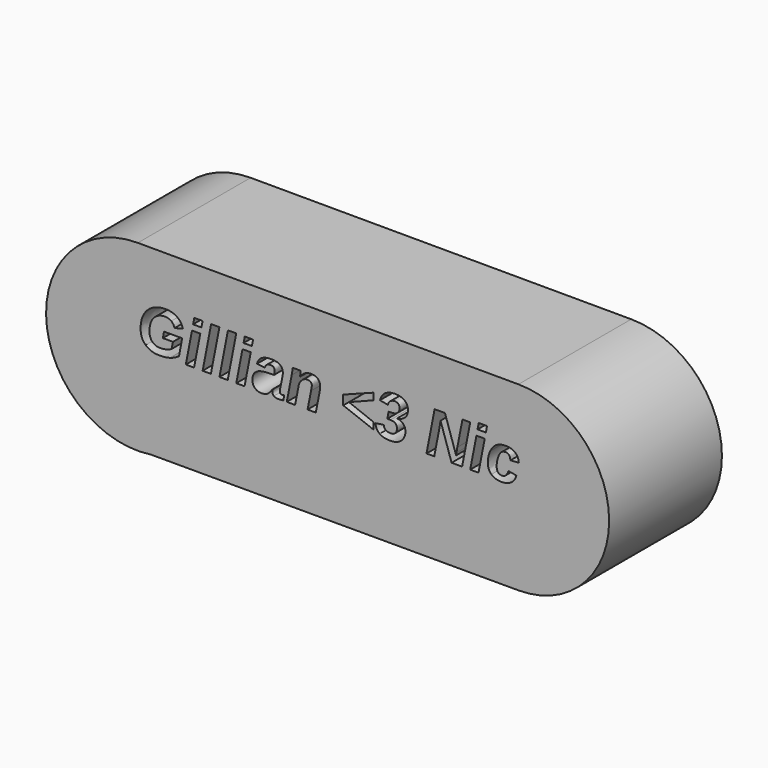
from build123d import *

# Parameters (mm, degrees)
F1_DEPTH = 25.4


with BuildPart() as f1:
    # F0 (on Front) → F1 (new body)
    with BuildSketch(Plane.XZ):
        with BuildLine():
            Line((28.869589976, 36.934029669), (-39.7119261324, 37.0742306113))
            ThreePointArc((-39.7119261324, 37.0742306113), (-56.2022137715, 19.4003067851), (-37.3673066497, 4.2496155947))
            Line((-37.3673066497, 4.2496155947), (28.869589976, 4.2496155947))
            ThreePointArc((28.869589976, 4.2496155947), (45.2117970132, 20.5918226319), (28.869589976, 36.934029669))
        make_face()
        with BuildLine():
            add(Edge.make_bspline(
                [(-33.9471180294, 20.7070778912), (-34.7784034926, 20.475170562), (-35.8015240626, 20.475170562)],
                knots=[0, 0, 0, 1, 1, 1], degree=2))
            add(Edge.make_bspline(
                [(-35.8015240626, 20.475170562), (-37.4010025537, 20.475170562), (-38.3064642581, 21.3192450322)],
                knots=[0, 0, 0, 1, 1, 1], degree=2))
            add(Edge.make_bspline(
                [(-38.3064642581, 21.3192450322), (-39.2119259626, 22.1633195025), (-39.2119259626, 23.6826535489)],
                knots=[0, 0, 0, 1, 1, 1], degree=2))
            add(Edge.make_bspline(
                [(-39.2119259626, 23.6826535489), (-39.2119259626, 25.0144154908), (-38.6551778524, 26.048619867)],
                knots=[0, 0, 0, 1, 1, 1], degree=2))
            add(Edge.make_bspline(
                [(-38.6551778524, 26.048619867), (-38.0984297422, 27.0828242432), (-37.0778669736, 27.6395723534)],
                knots=[0, 0, 0, 1, 1, 1], degree=2))
            add(Edge.make_bspline(
                [(-37.0778669736, 27.6395723534), (-36.0573042051, 28.1963204635), (-34.7255422631, 28.1963204635)],
                knots=[0, 0, 0, 1, 1, 1], degree=2))
            add(Edge.make_bspline(
                [(-34.7255422631, 28.1963204635), (-33.5114391867, 28.1963204635), (-32.6929427307, 27.6472457576)],
                knots=[0, 0, 0, 1, 1, 1], degree=2))
            add(Edge.make_bspline(
                [(-32.6929427307, 27.6472457576), (-31.8744462747, 27.0981710517), (-31.593088118, 26.1125649026)],
                knots=[0, 0, 0, 1, 1, 1], degree=2))
            Line((-31.593088118, 26.1125649026), (-33.0953701549, 25.6964958708))
            add(Edge.make_bspline(
                [(-33.0953701549, 25.6964958708), (-33.2505434414, 26.2984318062), (-33.6921904874, 26.6292407905)],
                knots=[0, 0, 0, 1, 1, 1], degree=2))
            add(Edge.make_bspline(
                [(-33.6921904874, 26.6292407905), (-34.1338375335, 26.9600497748), (-34.8108023106, 26.9600497748)],
                knots=[0, 0, 0, 1, 1, 1], degree=2))
            add(Edge.make_bspline(
                [(-34.8108023106, 26.9600497748), (-35.6582871828, 26.9600497748), (-36.297737539, 26.560180152)],
                knots=[0, 0, 0, 1, 1, 1], degree=2))
            add(Edge.make_bspline(
                [(-36.297737539, 26.560180152), (-36.9371878953, 26.1603105292), (-37.2782280853, 25.4253689198)],
                knots=[0, 0, 0, 1, 1, 1], degree=2))
            add(Edge.make_bspline(
                [(-37.2782280853, 25.4253689198), (-37.6192682753, 24.6904273103), (-37.6192682753, 23.7303991755)],
                knots=[0, 0, 0, 1, 1, 1], degree=2))
            add(Edge.make_bspline(
                [(-37.6192682753, 23.7303991755), (-37.6192682753, 22.7823074473), (-37.1102657917, 22.2409061457)],
                knots=[0, 0, 0, 1, 1, 1], degree=2))
            add(Edge.make_bspline(
                [(-37.1102657917, 22.2409061457), (-36.6012633081, 21.6995048441), (-35.6736339913, 21.6995048441)],
                knots=[0, 0, 0, 1, 1, 1], degree=2))
            add(Edge.make_bspline(
                [(-35.6736339913, 21.6995048441), (-35.0989812712, 21.6995048441), (-34.5550221681, 21.8384787215)],
                knots=[0, 0, 0, 1, 1, 1], degree=2))
            add(Edge.make_bspline(
                [(-34.5550221681, 21.8384787215), (-34.0110630651, 21.9774525989), (-33.6273928513, 22.2110651291)],
                knots=[0, 0, 0, 1, 1, 1], degree=2))
            Line((-33.6273928513, 22.2110651291), (-33.3835491155, 23.4268734064))
            Line((-33.3835491155, 23.4268734064), (-35.2047037301, 23.4268734064))
            Line((-35.2047037301, 23.4268734064), (-34.9983744151, 24.5352540239))
            Line((-34.9983744151, 24.5352540239), (-31.7260937921, 24.5352540239))
            Line((-31.7260937921, 24.5352540239), (-32.2853997037, 21.5085223377))
            add(Edge.make_bspline(
                [(-32.2853997037, 21.5085223377), (-33.1158325663, 20.9389852204), (-33.9471180294, 20.7070778912)],
                knots=[0, 0, 0, 1, 1, 1], degree=2))
        make_face(mode=Mode.SUBTRACT)
        Polygon((-29.579245796, 20.575777418), (-31.0712966273, 20.575777418), (-29.9509796031, 26.3410618299), (-28.453813169, 26.3410618299), align=None, mode=Mode.SUBTRACT)
        Polygon((-26.5473985069, 20.575777418), (-28.0394493382, 20.575777418), (-26.5047684832, 28.4844994241), (-25.0058968481, 28.4844994241), align=None, mode=Mode.SUBTRACT)
        Polygon((-20.4837039287, 20.575777418), (-21.97575476, 20.575777418), (-20.8554377358, 26.3410618299), (-19.3582713017, 26.3410618299), align=None, mode=Mode.SUBTRACT)
        Polygon((-23.5155512178, 20.575777418), (-25.0076020491, 20.575777418), (-23.4729211941, 28.4844994241), (-21.974049559, 28.4844994241), align=None, mode=Mode.SUBTRACT)
        with BuildLine():
            add(Edge.make_bspline(
                [(-13.9075964651, 20.5382629971), (-14.1369459929, 20.5229161886), (-14.3756741259, 20.5229161886)],
                knots=[0, 0, 0, 1, 1, 1], degree=2))
            add(Edge.make_bspline(
                [(-14.3756741259, 20.5229161886), (-14.9094020232, 20.5229161886), (-15.1967283833, 20.746297513)],
                knots=[0, 0, 0, 1, 1, 1], degree=2))
            add(Edge.make_bspline(
                [(-15.1967283833, 20.746297513), (-15.4840547434, 20.9696788375), (-15.4840547434, 21.3380022427)],
                knots=[0, 0, 0, 1, 1, 1], degree=2))
            add(Edge.make_bspline(
                [(-15.4840547434, 21.3380022427), (-15.4840547434, 21.5358055529), (-15.4584767291, 21.6790424327)],
                knots=[0, 0, 0, 1, 1, 1], degree=2))
            Line((-15.4584767291, 21.6790424327), (-15.4908755472, 21.6790424327))
            add(Edge.make_bspline(
                [(-15.4908755472, 21.6790424327), (-15.9376381961, 20.986730847), (-16.3750222397, 20.7275403026)],
                knots=[0, 0, 0, 1, 1, 1], degree=2))
            add(Edge.make_bspline(
                [(-16.3750222397, 20.7275403026), (-16.8124062834, 20.4683497582), (-17.439920233, 20.4683497582)],
                knots=[0, 0, 0, 1, 1, 1], degree=2))
            add(Edge.make_bspline(
                [(-17.439920233, 20.4683497582), (-18.1867982491, 20.4683497582), (-18.631855697, 20.9134072061)],
                knots=[0, 0, 0, 1, 1, 1], degree=2))
            add(Edge.make_bspline(
                [(-18.631855697, 20.9134072061), (-19.076913145, 21.3584646541), (-19.076913145, 22.0575970436)],
                knots=[0, 0, 0, 1, 1, 1], degree=2))
            add(Edge.make_bspline(
                [(-19.076913145, 22.0575970436), (-19.076913145, 23.0432031927), (-18.3973905664, 23.5470900734)],
                knots=[0, 0, 0, 1, 1, 1], degree=2))
            add(Edge.make_bspline(
                [(-18.3973905664, 23.5470900734), (-17.7178679878, 24.0509769541), (-16.1934183386, 24.0765549683)],
                knots=[0, 0, 0, 1, 1, 1], degree=2))
            Line((-16.1934183386, 24.0765549683), (-15.1754133714, 24.0936069778))
            add(Edge.make_bspline(
                [(-15.1754133714, 24.0936069778), (-15.0645753097, 24.598346459), (-15.0645753097, 24.7910341664)],
                knots=[0, 0, 0, 1, 1, 1], degree=2))
            add(Edge.make_bspline(
                [(-15.0645753097, 24.7910341664), (-15.0645753097, 25.4731145464), (-15.7398348859, 25.4731145464)],
                knots=[0, 0, 0, 1, 1, 1], degree=2))
            add(Edge.make_bspline(
                [(-15.7398348859, 25.4731145464), (-16.2411639652, 25.4731145464), (-16.486712902, 25.2787216381)],
                knots=[0, 0, 0, 1, 1, 1], degree=2))
            add(Edge.make_bspline(
                [(-16.486712902, 25.2787216381), (-16.7322618388, 25.0843287298), (-16.8226374891, 24.7160053246)],
                knots=[0, 0, 0, 1, 1, 1], degree=2))
            Line((-16.8226374891, 24.7160053246), (-18.22431267, 24.8814098167))
            add(Edge.make_bspline(
                [(-18.22431267, 24.8814098167), (-18.0418561683, 25.6487502442), (-17.405816214, 26.048619867)],
                knots=[0, 0, 0, 1, 1, 1], degree=2))
            add(Edge.make_bspline(
                [(-17.405816214, 26.048619867), (-16.7697762597, 26.4484894898), (-15.7142568716, 26.4484894898)],
                knots=[0, 0, 0, 1, 1, 1], degree=2))
            add(Edge.make_bspline(
                [(-15.7142568716, 26.4484894898), (-14.610991857, 26.4484894898), (-14.0968737705, 26.0597036732)],
                knots=[0, 0, 0, 1, 1, 1], degree=2))
            add(Edge.make_bspline(
                [(-14.0968737705, 26.0597036732), (-13.5827556841, 25.6709178566), (-13.5827556841, 24.8762942139)],
                knots=[0, 0, 0, 1, 1, 1], degree=2))
            add(Edge.make_bspline(
                [(-13.5827556841, 24.8762942139), (-13.5827556841, 24.6784909037), (-13.7106457554, 24.0390405474)],
                knots=[0, 0, 0, 1, 1, 1], degree=2))
            Line((-13.7106457554, 24.0390405474), (-14.0892003663, 22.1582038996))
            add(Edge.make_bspline(
                [(-14.0892003663, 22.1582038996), (-14.13183039, 21.9194757666), (-14.13183039, 21.7745336859)],
                knots=[0, 0, 0, 1, 1, 1], degree=2))
            add(Edge.make_bspline(
                [(-14.13183039, 21.7745336859), (-14.13183039, 21.6466436146), (-14.0781165601, 21.5775829761)],
                knots=[0, 0, 0, 1, 1, 1], degree=2))
            add(Edge.make_bspline(
                [(-14.0781165601, 21.5775829761), (-14.0244027302, 21.5085223377), (-13.9553420917, 21.4761235196)],
                knots=[0, 0, 0, 1, 1, 1], degree=2))
            add(Edge.make_bspline(
                [(-13.9553420917, 21.4761235196), (-13.8862814532, 21.4437247016), (-13.8172208147, 21.4360512973)],
                knots=[0, 0, 0, 1, 1, 1], degree=2))
            add(Edge.make_bspline(
                [(-13.8172208147, 21.4360512973), (-13.7481601763, 21.428377893), (-13.7106457554, 21.428377893)],
                knots=[0, 0, 0, 1, 1, 1], degree=2))
            add(Edge.make_bspline(
                [(-13.7106457554, 21.428377893), (-13.5503568661, 21.428377893), (-13.3798367711, 21.4658923139)],
                knots=[0, 0, 0, 1, 1, 1], degree=2))
            Line((-13.3798367711, 21.4658923139), (-13.4548656129, 20.6405750541))
            add(Edge.make_bspline(
                [(-13.4548656129, 20.6405750541), (-13.6782469373, 20.5536098057), (-13.9075964651, 20.5382629971)],
                knots=[0, 0, 0, 1, 1, 1], degree=2))
        make_face(mode=Mode.SUBTRACT)
        with BuildLine():
            Line((-7.6418355743, 20.575777418), (-9.1287708027, 20.575777418))
            Line((-9.1287708027, 20.575777418), (-8.4995516522, 23.7457459841))
            add(Edge.make_bspline(
                [(-8.4995516522, 23.7457459841), (-8.3614303752, 24.4073639526), (-8.3614303752, 24.6256296742)],
                knots=[0, 0, 0, 1, 1, 1], degree=2))
            add(Edge.make_bspline(
                [(-8.3614303752, 24.6256296742), (-8.3614303752, 25.3128256571), (-9.1714008265, 25.3128256571)],
                knots=[0, 0, 0, 1, 1, 1], degree=2))
            add(Edge.make_bspline(
                [(-9.1714008265, 25.3128256571), (-9.7085391257, 25.3128256571), (-10.1672381813, 24.8762942139)],
                knots=[0, 0, 0, 1, 1, 1], degree=2))
            add(Edge.make_bspline(
                [(-10.1672381813, 24.8762942139), (-10.6259372368, 24.4397627707), (-10.7435961024, 23.8054280173)],
                knots=[0, 0, 0, 1, 1, 1], degree=2))
            Line((-10.7435961024, 23.8054280173), (-11.371110052, 20.575777418))
            Line((-11.371110052, 20.575777418), (-12.8750972899, 20.575777418))
            Line((-12.8750972899, 20.575777418), (-11.9900979968, 25.109906744))
            add(Edge.make_bspline(
                [(-11.9900979968, 25.109906744), (-11.9048379493, 25.5310913787), (-11.7871790838, 26.3410618299)],
                knots=[0, 0, 0, 1, 1, 1], degree=2))
            Line((-11.7871790838, 26.3410618299), (-10.3599258886, 26.3410618299))
            add(Edge.make_bspline(
                [(-10.3599258886, 26.3410618299), (-10.3599258886, 26.2933162033), (-10.4102293166, 25.8934465806)],
                knots=[0, 0, 0, 1, 1, 1], degree=2))
            add(Edge.make_bspline(
                [(-10.4102293166, 25.8934465806), (-10.4605327447, 25.4935769578), (-10.4878159599, 25.3554556808)],
                knots=[0, 0, 0, 1, 1, 1], degree=2))
            Line((-10.4878159599, 25.3554556808), (-10.4707639504, 25.3554556808))
            add(Edge.make_bspline(
                [(-10.4707639504, 25.3554556808), (-10.0717469281, 25.9096459896), (-9.5891750592, 26.1765099383)],
                knots=[0, 0, 0, 1, 1, 1], degree=2))
            add(Edge.make_bspline(
                [(-9.5891750592, 26.1765099383), (-9.1066031904, 26.4433738869), (-8.4842048436, 26.4433738869)],
                knots=[0, 0, 0, 1, 1, 1], degree=2))
            add(Edge.make_bspline(
                [(-8.4842048436, 26.4433738869), (-7.6742343924, 26.4433738869), (-7.2632809634, 26.0537354699)],
                knots=[0, 0, 0, 1, 1, 1], degree=2))
            add(Edge.make_bspline(
                [(-7.2632809634, 26.0537354699), (-6.8523275345, 25.6640970528), (-6.8523275345, 24.9291554433)],
                knots=[0, 0, 0, 1, 1, 1], degree=2))
            add(Edge.make_bspline(
                [(-6.8523275345, 24.9291554433), (-6.8523275345, 24.7961497692), (-6.8898419554, 24.5054130073)],
                knots=[0, 0, 0, 1, 1, 1], degree=2))
            add(Edge.make_bspline(
                [(-6.8898419554, 24.5054130073), (-6.9273563763, 24.2146762453), (-6.9648707972, 24.0560925569)],
                knots=[0, 0, 0, 1, 1, 1], degree=2))
            Line((-6.9648707972, 24.0560925569), (-7.6418355743, 20.575777418))
        make_face(mode=Mode.SUBTRACT)
        Polygon((-28.2577150598, 27.3812344094), (-29.7548814939, 27.3812344094), (-29.5366157723, 28.4844994241), (-28.0377441372, 28.4844994241), align=None, mode=Mode.SUBTRACT)
        Polygon((-19.1621731925, 27.3812344094), (-20.6593396266, 27.3812344094), (-20.441073905, 28.4844994241), (-18.9422022699, 28.4844994241), align=None, mode=Mode.SUBTRACT)
        Polygon((2.7701214264, 21.2425109895), (-2.7018684222, 23.3262665504), (-2.7018684222, 25.041698706), (2.7701214264, 27.1254542669), (2.7701214264, 25.9096459896), (-1.6685166465, 24.1788670253), (2.7701214264, 22.451498463), align=None, mode=Mode.SUBTRACT)
        with BuildLine():
            Line((5.4728649321, 24.9939530794), (5.8616507487, 24.9939530794))
            add(Edge.make_bspline(
                [(5.8616507487, 24.9939530794), (6.6562743914, 24.9939530794), (7.0476180094, 25.3025944514)],
                knots=[0, 0, 0, 1, 1, 1], degree=2))
            add(Edge.make_bspline(
                [(7.0476180094, 25.3025944514), (7.4389616275, 25.6112358233), (7.4389616275, 26.1756573378)],
                knots=[0, 0, 0, 1, 1, 1], degree=2))
            add(Edge.make_bspline(
                [(7.4389616275, 26.1756573378), (7.4389616275, 26.5593275515), (7.233484913, 26.781003675)],
                knots=[0, 0, 0, 1, 1, 1], degree=2))
            add(Edge.make_bspline(
                [(7.233484913, 26.781003675), (7.0280081985, 27.0026797985), (6.601707961, 27.0026797985)],
                knots=[0, 0, 0, 1, 1, 1], degree=2))
            add(Edge.make_bspline(
                [(6.601707961, 27.0026797985), (5.6109862091, 27.0026797985), (5.339859258, 26.0221892523)],
                knots=[0, 0, 0, 1, 1, 1], degree=2))
            Line((5.339859258, 26.0221892523), (3.9160164648, 26.2984318062))
            add(Edge.make_bspline(
                [(3.9160164648, 26.2984318062), (4.4599755678, 28.1963204635), (6.6613899943, 28.1963204635)],
                knots=[0, 0, 0, 1, 1, 1], degree=2))
            add(Edge.make_bspline(
                [(6.6613899943, 28.1963204635), (7.7424873965, 28.1963204635), (8.3503915352, 27.7111907933)],
                knots=[0, 0, 0, 1, 1, 1], degree=2))
            add(Edge.make_bspline(
                [(8.3503915352, 27.7111907933), (8.9582956739, 27.226061123), (8.9582956739, 26.3632294423)],
                knots=[0, 0, 0, 1, 1, 1], degree=2))
            add(Edge.make_bspline(
                [(8.9582956739, 26.3632294423), (8.9582956739, 25.5310913787), (8.4407671856, 25.025499297)],
                knots=[0, 0, 0, 1, 1, 1], degree=2))
            add(Edge.make_bspline(
                [(8.4407671856, 25.025499297), (7.9232386972, 24.5199072153), (7.0331238014, 24.4397627707)],
                knots=[0, 0, 0, 1, 1, 1], degree=2))
            Line((7.0331238014, 24.4397627707), (7.0280081985, 24.4175951583))
            add(Edge.make_bspline(
                [(7.0280081985, 24.4175951583), (7.7476029994, 24.3067570966), (8.1235998089, 23.8881302634)],
                knots=[0, 0, 0, 1, 1, 1], degree=2))
            add(Edge.make_bspline(
                [(8.1235998089, 23.8881302634), (8.4995966183, 23.4695034302), (8.4995966183, 22.8027698587)],
                knots=[0, 0, 0, 1, 1, 1], degree=2))
            add(Edge.make_bspline(
                [(8.4995966183, 22.8027698587), (8.4995966183, 22.1428570911), (8.1534408255, 21.6014557894)],
                knots=[0, 0, 0, 1, 1, 1], degree=2))
            add(Edge.make_bspline(
                [(8.1534408255, 21.6014557894), (7.8072850326, 21.0600544878), (7.1780658821, 20.764202123)],
                knots=[0, 0, 0, 1, 1, 1], degree=2))
            add(Edge.make_bspline(
                [(7.1780658821, 20.764202123), (6.5488467316, 20.4683497582), (5.7337606775, 20.4683497582)],
                knots=[0, 0, 0, 1, 1, 1], degree=2))
            add(Edge.make_bspline(
                [(5.7337606775, 20.4683497582), (4.5298888068, 20.4683497582), (3.855481831, 20.9645632346)],
                knots=[0, 0, 0, 1, 1, 1], degree=2))
            add(Edge.make_bspline(
                [(3.855481831, 20.9645632346), (3.1810748553, 21.4607767111), (3.0958148078, 22.4037528364)],
                knots=[0, 0, 0, 1, 1, 1], degree=2))
            Line((3.0958148078, 22.4037528364), (4.5980968448, 22.6066717495))
            add(Edge.make_bspline(
                [(4.5980968448, 22.6066717495), (4.657778878, 22.1258050816), (4.9348740324, 21.8998659557)],
                knots=[0, 0, 0, 1, 1, 1], degree=2))
            add(Edge.make_bspline(
                [(4.9348740324, 21.8998659557), (5.2119691868, 21.6739268298), (5.8036739164, 21.6739268298)],
                knots=[0, 0, 0, 1, 1, 1], degree=2))
            add(Edge.make_bspline(
                [(5.8036739164, 21.6739268298), (6.3578642252, 21.6739268298), (6.6690633985, 21.9723369961)],
                knots=[0, 0, 0, 1, 1, 1], degree=2))
            add(Edge.make_bspline(
                [(6.6690633985, 21.9723369961), (6.9802625719, 22.2707471623), (6.9802625719, 22.792538653)],
                knots=[0, 0, 0, 1, 1, 1], degree=2))
            add(Edge.make_bspline(
                [(6.9802625719, 22.792538653), (6.9802625719, 23.783260405), (5.8087895193, 23.783260405)],
                knots=[0, 0, 0, 1, 1, 1], degree=2))
            Line((5.8087895193, 23.783260405), (5.237547201, 23.783260405))
            Line((5.237547201, 23.783260405), (5.4728649321, 24.9939530794))
        make_face(mode=Mode.SUBTRACT)
        with BuildLine():
            Line((18.7188659117, 20.575777418), (16.8226824553, 20.575777418))
            Line((16.8226824553, 20.575777418), (14.8293025447, 26.6019575753))
            add(Edge.make_bspline(
                [(14.8293025447, 26.6019575753), (14.7065280763, 25.7391258946), (14.6263836317, 25.3298776666)],
                knots=[0, 0, 0, 1, 1, 1], degree=2))
            Line((14.6263836317, 25.3298776666), (13.6987543149, 20.575777418))
            Line((13.6987543149, 20.575777418), (12.3038999378, 20.575777418))
            Line((12.3038999378, 20.575777418), (13.763551951, 28.0837772008))
            Line((13.763551951, 28.0837772008), (15.6290417903, 28.0837772008))
            Line((15.6290417903, 28.0837772008), (17.6377685094, 22.0047358141))
            Line((17.6377685094, 22.0047358141), (17.7008609445, 22.4412672573))
            add(Edge.make_bspline(
                [(17.7008609445, 22.4412672573), (17.7605429778, 22.8829143034), (17.856034231, 23.3688965741)],
                knots=[0, 0, 0, 1, 1, 1], degree=2))
            Line((17.856034231, 23.3688965741), (18.7836635478, 28.0837772008))
            Line((18.7836635478, 28.0837772008), (20.1785179249, 28.0837772008))
            Line((20.1785179249, 28.0837772008), (18.7188659117, 20.575777418))
        make_face(mode=Mode.SUBTRACT)
        Polygon((21.6705687561, 20.575777418), (20.1785179249, 20.575777418), (21.298834949, 26.3410618299), (22.7960013831, 26.3410618299), align=None, mode=Mode.SUBTRACT)
        with BuildLine():
            add(Edge.make_bspline(
                [(24.9326181735, 22.7447930264), (24.9326181735, 21.498291132), (25.8807099017, 21.498291132)],
                knots=[0, 0, 0, 1, 1, 1], degree=2))
            add(Edge.make_bspline(
                [(25.8807099017, 21.498291132), (26.3223569477, 21.498291132), (26.6105359083, 21.7779440878)],
                knots=[0, 0, 0, 1, 1, 1], degree=2))
            add(Edge.make_bspline(
                [(26.6105359083, 21.7779440878), (26.8987148688, 22.0575970436), (27.0692349638, 22.6066717495)],
                knots=[0, 0, 0, 1, 1, 1], degree=2))
            Line((27.0692349638, 22.6066717495), (28.5135401685, 22.3389552003))
            add(Edge.make_bspline(
                [(28.5135401685, 22.3389552003), (27.9422978502, 20.4683497582), (25.7954498542, 20.4683497582)],
                knots=[0, 0, 0, 1, 1, 1], degree=2))
            add(Edge.make_bspline(
                [(25.7954498542, 20.4683497582), (24.6239768015, 20.4683497582), (23.9921998495, 21.0685804926)],
                knots=[0, 0, 0, 1, 1, 1], degree=2))
            add(Edge.make_bspline(
                [(23.9921998495, 21.0685804926), (23.3604228976, 21.668811227), (23.3604228976, 22.7345618207)],
                knots=[0, 0, 0, 1, 1, 1], degree=2))
            add(Edge.make_bspline(
                [(23.3604228976, 22.7345618207), (23.3604228976, 23.7730291993), (23.7816075322, 24.684459107)],
                knots=[0, 0, 0, 1, 1, 1], degree=2))
            add(Edge.make_bspline(
                [(23.7816075322, 24.684459107), (24.2027921669, 25.5958890148), (24.9036297573, 26.0221892523)],
                knots=[0, 0, 0, 1, 1, 1], degree=2))
            add(Edge.make_bspline(
                [(24.9036297573, 26.0221892523), (25.6044673478, 26.4484894898), (26.6480503292, 26.4484894898)],
                knots=[0, 0, 0, 1, 1, 1], degree=2))
            add(Edge.make_bspline(
                [(26.6480503292, 26.4484894898), (27.6558240906, 26.4484894898), (28.257760026, 25.9394870062)],
                knots=[0, 0, 0, 1, 1, 1], degree=2))
            add(Edge.make_bspline(
                [(28.257760026, 25.9394870062), (28.8596959613, 25.4304845226), (28.9347248031, 24.5250228182)],
                knots=[0, 0, 0, 1, 1, 1], degree=2))
            Line((28.9347248031, 24.5250228182), (27.4205063595, 24.4022483498))
            add(Edge.make_bspline(
                [(27.4205063595, 24.4022483498), (27.3625295272, 25.4202533169), (26.5303914636, 25.4202533169)],
                knots=[0, 0, 0, 1, 1, 1], degree=2))
            add(Edge.make_bspline(
                [(26.5303914636, 25.4202533169), (25.9608543463, 25.4202533169), (25.6385713668, 25.0280570984)],
                knots=[0, 0, 0, 1, 1, 1], degree=2))
            add(Edge.make_bspline(
                [(25.6385713668, 25.0280570984), (25.3162883872, 24.6358608799), (25.0553926419, 23.6400235252)],
                knots=[0, 0, 0, 1, 1, 1], degree=2))
            add(Edge.make_bspline(
                [(25.0553926419, 23.6400235252), (24.9326181735, 23.0278563841), (24.9326181735, 22.7447930264)],
                knots=[0, 0, 0, 1, 1, 1], degree=2))
        make_face(mode=Mode.SUBTRACT)
        Polygon((22.9920994924, 27.3812344094), (21.4949330583, 27.3812344094), (21.7131987799, 28.4844994241), (23.2120704149, 28.4844994241), align=None, mode=Mode.SUBTRACT)
    extrude(amount=F1_DEPTH)


solid = f1.part
